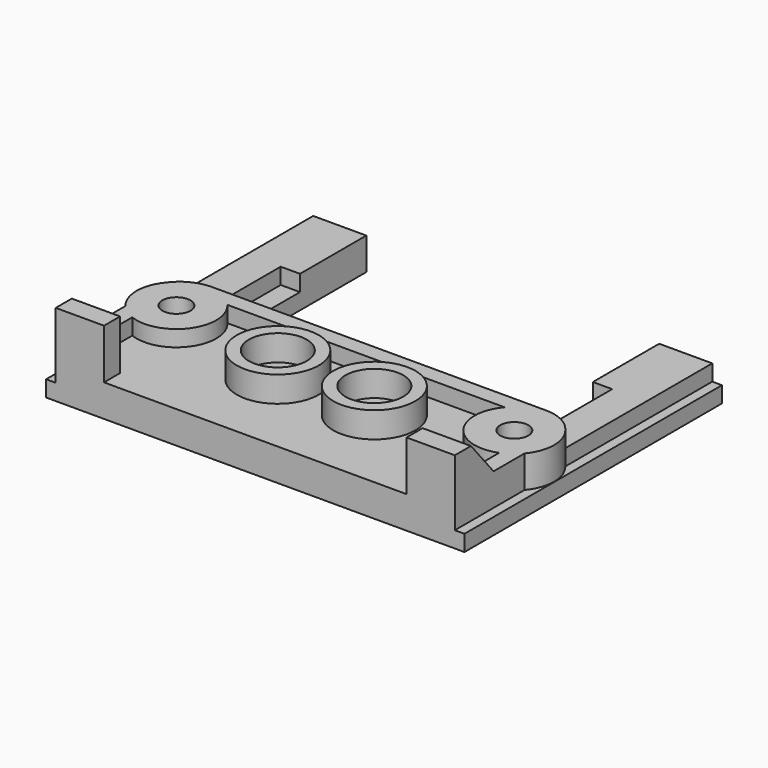
from build123d import *

# Parameters (mm, degrees)
F1_DEPTH     = 2
F2_W         = 0.6
F2_H         = 20
F3_DEPTH     = 1
F5_DEPTH     = 1
F6_W         = 3
F6_H         = 1.25
F7_DEPTH     = 3.1
F8_W         = 1
F8_H         = 1.75
F9_DEPTH     = 2.1
F10_SIZE2    = 2.085568787
F10_SIZE     = 1.75
F11_R        = 2.475
F11_R_2      = 0.875
F12_DEPTH    = 3
F13_T1_DEPTH = 6.0259261824
F14_R        = 0.875
F15_DEPTH    = 5.101
F17_DEPTH    = 1
F18_W        = 5.15
F18_H        = 1
F19_DEPTH    = 1.2
F20_R        = 1.6
F21_DEPTH    = 2
F22_R        = 2.55
F22_R_2      = 1.8
F23_DEPTH    = 1.6


# Not quite as in the source:
# - a fillet or chamfer that OpenCascade refuses, or shapes differently, is made with other operations: its cross-section is extruded or revolved along the edge and cut away or added


with BuildPart() as f1:
    # F0 (on Top) → F1 (new body)
    with BuildSketch(Plane.XY):
        Polygon((0, 3.8), (0, -7), (13, -7), (13, 13), (9.1, 13), (9.1, 3.8), align=None)
    extrude(amount=F1_DEPTH)

    # F2 (on face) → F3 (cut)
    with BuildSketch(Plane.XY.offset(2)):
        with Locations((12.7, 3)):
            Rectangle(F2_W, F2_H)
    extrude(amount=-F3_DEPTH, mode=Mode.SUBTRACT)

    # F4 (on face) → F5 (join)
    with BuildSketch(Plane.XY.offset(2)):
        Polygon((12.4, -7), (12.4, 2.6), (0, 2.6), (0, 1.6), (11.4, 1.6), (11.4, -7), align=None)
    extrude(amount=F5_DEPTH)

    # F6 (on face) → F7 (join)
    with BuildSketch(Plane.XY.offset(2)):
        with Locations((10.9, -6.375)):
            Rectangle(F6_W, F6_H)
    extrude(amount=F7_DEPTH)

    # F8 (on face) → F9 (join)
    with BuildSketch(Plane.XY.offset(3)):
        with Locations((11.9, -4.875)):
            Rectangle(F8_W, F8_H)
    extrude(amount=F9_DEPTH)

    # F10
    f10_edges = [f1.edges().sort_by_distance(p)[0] for p in [
        (11.9, -4, 5.1),
    ]]
    f10_side = f1.faces().sort_by_distance((11.218182, -5.897727, 5.1))[0]
    chamfer(f10_edges, length=F10_SIZE, length2=F10_SIZE2, reference=f10_side)

    # F11 (on Top) → F12 (join)
    with BuildSketch(Plane.XY):
        with Locations((10.5, 0)):
            Circle(F11_R)
        with Locations((10.5, 0)):
            Circle(F11_R_2, mode=Mode.SUBTRACT)
    extrude(amount=F12_DEPTH)

    # F13: fillet of radius 2.5 on 1 edges, made by hand

    # F13_s2 → F13_t1 (cut)
    with BuildSketch(Plane.XY.offset(2)):
        with BuildLine():
            ThreePointArc((12.4, 1.5860721926), (11.515422474, 2.3321716423), (10.389629527, 2.6))
            Line((10.389629527, 2.6), (12.4, 2.6))
            Line((12.4, 2.6), (12.4, 1.5860721926))
        make_face()
    extrude(amount=F13_T1_DEPTH, mode=Mode.SUBTRACT)

    # F14 (on face) → F15 (cut, through all)
    with BuildSketch(Plane.XY):
        with Locations((10.5, 0)):
            Circle(F14_R)
    extrude(amount=F15_DEPTH, mode=Mode.SUBTRACT)

    # F16 (on face) → F17 (cut)
    with BuildSketch(Plane.XY.offset(2)):
        Polygon((10.3, 13), (9.1, 13), (9.1, 3.8), (0, 3.8), (0, 2.6), (10.3, 2.6), align=None)
    extrude(amount=-F17_DEPTH, mode=Mode.SUBTRACT)

    # F18 (on face) → F19 (join)
    with BuildSketch(Plane(origin=(10.3, 0, 0), x_dir=(0, -1, 0), z_dir=(-1, 0, 0))):
        with Locations((-10.425, 1.5)):
            Rectangle(F18_W, F18_H)
    extrude(amount=F19_DEPTH)

    # F20 (on face) → F21 (cut)
    with BuildSketch(Plane.XY):
        with Locations((10.5, 0)):
            Circle(F20_R)
    extrude(amount=F21_DEPTH, mode=Mode.SUBTRACT)

    # F22 (on face) → F23 (join)
    with BuildSketch(Plane.XY.offset(2)):
        with Locations((3, -1.5)):
            Circle(F22_R)
        with Locations((3, -1.5)):
            Circle(F22_R_2, mode=Mode.SUBTRACT)
    extrude(amount=F23_DEPTH)

    # F24: F1 across face


with BuildPart() as f1_1:
    add(f1.part)
    add(f1.part.mirror(Plane(origin=(0, -1.6962616822, 1.0420560748), x_dir=(0, -1, 0), z_dir=(-1, 0, 0))))


solid = f1_1.part
